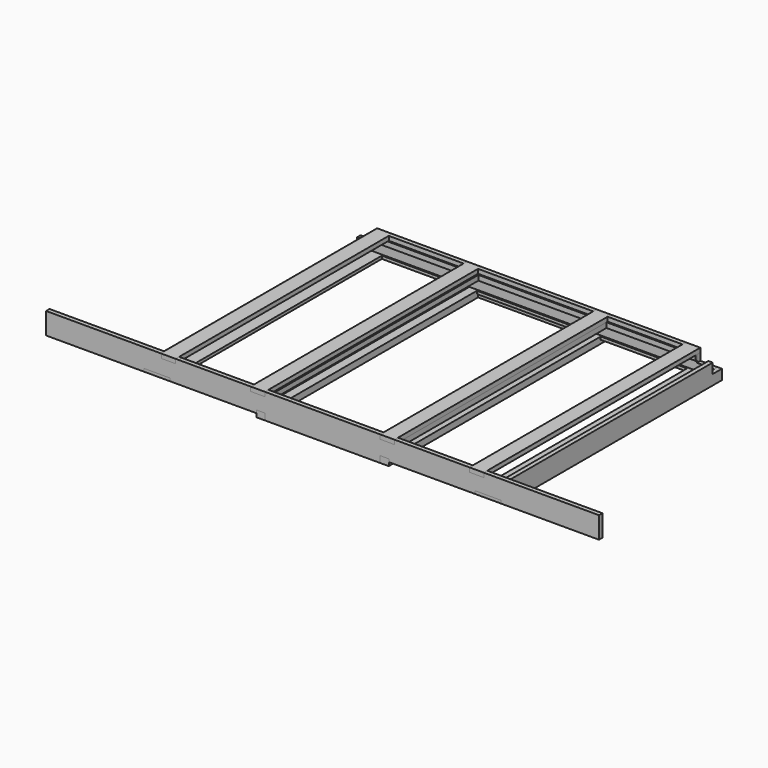
from build123d import *

# Parameters (mm, degrees)
F0_W      = 254
F0_H      = 15.875
F1_DEPTH  = 19.05
F2_W      = 381
F2_H      = 12.7
F3_DEPTH  = 6.35
F2_W_2    = 508
F5_DEPTH  = 6.35
F6_W      = 63.5
F6_H      = 19.05
F7_DEPTH  = 1193.8
F6_W_2    = 114.3
F6_H_2    = 12.7
F6_W_3    = 38.1
F6_H_3    = 28.575
F9_DEPTH  = 19.05
F10_W     = 1955.8
F10_H     = 22.225
F11_DEPTH = 6.35
F12_W     = 381
F12_H     = 12.7
F13_DEPTH = 6.35
F12_W_2   = 508
F14_W     = 69.85
F14_H     = 1143
F15_DEPTH = 22.225
F16_W     = 69.85
F16_H     = 1143
F17_DEPTH = 22.225
F18_W     = 1168.4
F18_H     = 19.05
F19_DEPTH = 3.175
F21_DEPTH = 19.05


# Not quite as in the source:
# - a feature names something its author has since deleted; it is built from what else it names


with BuildPart() as f1:
    # F0 (on Front) → F1 (new body)
    with BuildSketch(Plane.XZ):
        Polygon((114.3, 12.7), (114.3, 0), (495.3, 0), (495.3, 12.7), (533.4, 12.7), (533.4, 0), (787.4, 0), (787.4, 95.25), (533.4, 95.25), (533.4, 76.2), (469.9, 76.2), (469.9, 95.25), (139.7, 95.25), (139.7, 76.2), (76.2, 76.2), (76.2, 44.45), (0, 44.45), (0, 12.7), align=None)
        Polygon((787.4, 95.25), (787.4, 0), (1041.4, 0), (1041.4, 12.7), (1079.5, 12.7), (1079.5, 0), (1460.5, 0), (1460.5, 12.7), (1574.8, 12.7), (1574.8, 44.45), (1498.6, 44.45), (1498.6, 76.2), (1435.1, 76.2), (1435.1, 95.25), (1104.9, 95.25), (1104.9, 76.2), (1041.4, 76.2), (1041.4, 95.25), align=None)
        with Locations((660.4, -7.9375)):
            Rectangle(F0_W, F0_H)
        with Locations((914.4, -7.9375)):
            Rectangle(F0_W, F0_H)
    extrude(amount=F1_DEPTH)


with BuildPart() as f3:
    # F2 (on face) → F3 (new body)
    with BuildSketch(Plane.XZ.offset(19.05)):
        with Locations((304.8, 6.35)):
            Rectangle(F2_W, F2_H)
    extrude(amount=F3_DEPTH)


with BuildPart() as f3b:
    # F2 (on face) → F3, piece 2 (new body)
    with BuildSketch(Plane.XZ.offset(19.05)):
        with Locations((1270, 6.35)):
            Rectangle(F2_W, F2_H)
    extrude(amount=F3_DEPTH)


with BuildPart() as f3c:
    # F2 (on face) → F3, piece 3 (new body)
    with BuildSketch(Plane.XZ.offset(19.05)):
        with Locations((787.4, 6.35)):
            Rectangle(F2_W_2, F2_H)
    extrude(amount=F3_DEPTH)


with BuildPart() as f5:
    # F4 (on face) → F5 (new body)
    with BuildSketch(Plane.XZ.offset(19.05)):
        Polygon((76.2, 76.2), (76.2, 53.975), (1498.6, 53.975), (1498.6, 76.2), (1435.1, 76.2), (1104.9, 76.2), (1041.4, 76.2), (533.4, 76.2), (469.9, 76.2), (139.7, 76.2), align=None)
    extrude(amount=F5_DEPTH)


with BuildPart() as f7:
    # F6 (on Front) → F7 (new body)
    with BuildSketch(Plane.XZ):
        with Locations((107.95, 85.725)):
            Rectangle(F6_W, F6_H)
    extrude(amount=F7_DEPTH)


with BuildPart() as f7b:
    # F6 (on Front) → F7, piece 2 (new body)
    with BuildSketch(Plane.XZ):
        with Locations((501.65, 85.725)):
            Rectangle(F6_W, F6_H)
    extrude(amount=F7_DEPTH)


with BuildPart() as f7c:
    # F6 (on Front) → F7, piece 3 (new body)
    with BuildSketch(Plane.XZ):
        with Locations((1466.85, 85.725)):
            Rectangle(F6_W, F6_H)
    extrude(amount=F7_DEPTH)


with BuildPart() as f7d:
    # F6 (on Front) → F7, piece 4 (new body)
    with BuildSketch(Plane.XZ):
        with Locations((1073.15, 85.725)):
            Rectangle(F6_W, F6_H)
    extrude(amount=F7_DEPTH)


with BuildPart() as f7e:
    # F6 (on Front) → F7, piece 5 (new body)
    with BuildSketch(Plane.XZ):
        with Locations((1517.65, 6.35)):
            Rectangle(F6_W_2, F6_H_2)
    extrude(amount=F7_DEPTH)


with BuildPart() as f7f:
    # F6 (on Front) → F7, piece 6 (new body)
    with BuildSketch(Plane.XZ):
        with Locations((57.15, 6.35)):
            Rectangle(F6_W_2, F6_H_2)
    extrude(amount=F7_DEPTH)


with BuildPart() as f7g:
    # F6 (on Front) → F7, piece 7 (new body)
    with BuildSketch(Plane.XZ):
        with Locations((514.35, -1.5875)):
            Rectangle(F6_W_3, F6_H_3)
    extrude(amount=F7_DEPTH)


with BuildPart() as f7h:
    # F6 (on Front) → F7, piece 8 (new body)
    with BuildSketch(Plane.XZ):
        with Locations((1060.45, -1.5875)):
            Rectangle(F6_W_3, F6_H_3)
    extrude(amount=F7_DEPTH)


with BuildPart() as f9:
    # F8 (on face) → F9 (new body)
    with BuildSketch(Plane.XZ.offset(1193.8)):
        Polygon((469.9, 95.25), (292.1, 95.25), (139.7, 95.25), (139.7, 76.2), (76.2, 76.2), (76.2, 95.25), (-431.8, 95.25), (-431.8, 0), (0, 0), (0, 12.7), (114.3, 12.7), (114.3, 0), (317.5, 0), (495.3, 0), (495.3, 12.7), (533.4, 12.7), (533.4, 0), (787.4, 0), (787.4, 95.25), (533.4, 95.25), (533.4, 76.2), (469.9, 76.2), align=None)
        Polygon((1041.4, 95.25), (787.4, 95.25), (787.4, 0), (1041.4, 0), (1041.4, 12.7), (1079.5, 12.7), (1079.5, 0), (1257.3, 0), (1460.5, 0), (1460.5, 12.7), (1574.8, 12.7), (1574.8, 0), (2006.6, 0), (2006.6, 95.25), (1498.6, 95.25), (1498.6, 76.2), (1435.1, 76.2), (1435.1, 95.25), (1282.7, 95.25), (1104.9, 95.25), (1104.9, 76.2), (1041.4, 76.2), align=None)
        Polygon((1041.4, 0), (787.4, 0), (533.4, 0), (533.4, -15.875), (1041.4, -15.875), align=None)
    extrude(amount=-F9_DEPTH)


with BuildPart() as f11:
    # F10 (on face) → F11 (new body)
    with BuildSketch(Plane(origin=(0, -1174.75, 0), x_dir=(-1, 0, 0), z_dir=(0, 1, 0))):
        with Locations((-546.1, 65.0875)):
            Rectangle(F10_W, F10_H)
    extrude(amount=F11_DEPTH)


with BuildPart() as f13:
    # F12 (on face) → F13 (new body)
    with BuildSketch(Plane(origin=(0, -1174.75, 0), x_dir=(-1, 0, 0), z_dir=(0, 1, 0))):
        with Locations((-1270, 6.35)):
            Rectangle(F12_W, F12_H)
    extrude(amount=F13_DEPTH)


with BuildPart() as f13b:
    # F12 (on face) → F13, piece 2 (new body)
    with BuildSketch(Plane(origin=(0, -1174.75, 0), x_dir=(-1, 0, 0), z_dir=(0, 1, 0))):
        with Locations((-304.8, 6.35)):
            Rectangle(F12_W, F12_H)
    extrude(amount=F13_DEPTH)


with BuildPart() as f13c:
    # F12 (on face) → F13, piece 3 (new body)
    with BuildSketch(Plane(origin=(0, -1174.75, 0), x_dir=(-1, 0, 0), z_dir=(0, 1, 0))):
        with Locations((-787.4, 6.35)):
            Rectangle(F12_W_2, F12_H)
    extrude(amount=F13_DEPTH)


with BuildPart() as f15:
    # F14 (on face) → F15 (new body)
    with BuildSketch(Plane(origin=(0, 0, 76.2), x_dir=(1, 0, 0), z_dir=(0, 0, -1))):
        with Locations((1069.975, 596.9)):
            Rectangle(F14_W, F14_H)
    extrude(amount=F15_DEPTH)


with BuildPart() as f17:
    # F16 (on face) → F17 (new body)
    with BuildSketch(Plane(origin=(0, 0, 76.2), x_dir=(1, 0, 0), z_dir=(0, 0, -1))):
        with Locations((504.825, 596.9)):
            Rectangle(F16_W, F16_H)
    extrude(amount=F17_DEPTH)


with BuildPart() as f19:
    # F18 (on face) → F19 (new body)
    with BuildSketch(Plane(origin=(76.2, 0, 0), x_dir=(0, -1, 0), z_dir=(-1, 0, 0))):
        with Locations((584.2, 66.675)):
            Rectangle(F18_W, F18_H)
        Polygon((1174.75, 76.2), (1174.75, 95.25), (0, 95.25), (0, 76.2), (1168.4, 76.2), align=None)
    extrude(amount=F19_DEPTH)


with BuildPart() as f21:
    # F20 (on face) → F21 (new body)
    with BuildSketch(Plane.YZ.offset(1574.8)):
        Polygon((-1162.05, 12.7), (-1174.75, 12.7), (-1174.75, 0), (0, 0), (0, 12.7), align=None)
        Polygon((-50.8, 88.9), (-1174.75, 88.9), (-1174.75, 57.15), (-1162.05, 57.15), (-1162.05, 12.7), (0, 12.7), (0, 44.45), (-50.8, 44.45), align=None)
    extrude(amount=F21_DEPTH)


solid = Compound([f1.part, f3.part, f3b.part, f3c.part, f5.part, f7.part, f7b.part, f7c.part, f7d.part, f7e.part, f7f.part, f7g.part, f7h.part, f9.part, f11.part, f13.part, f13b.part, f13c.part, f15.part, f17.part, f19.part, f21.part])
